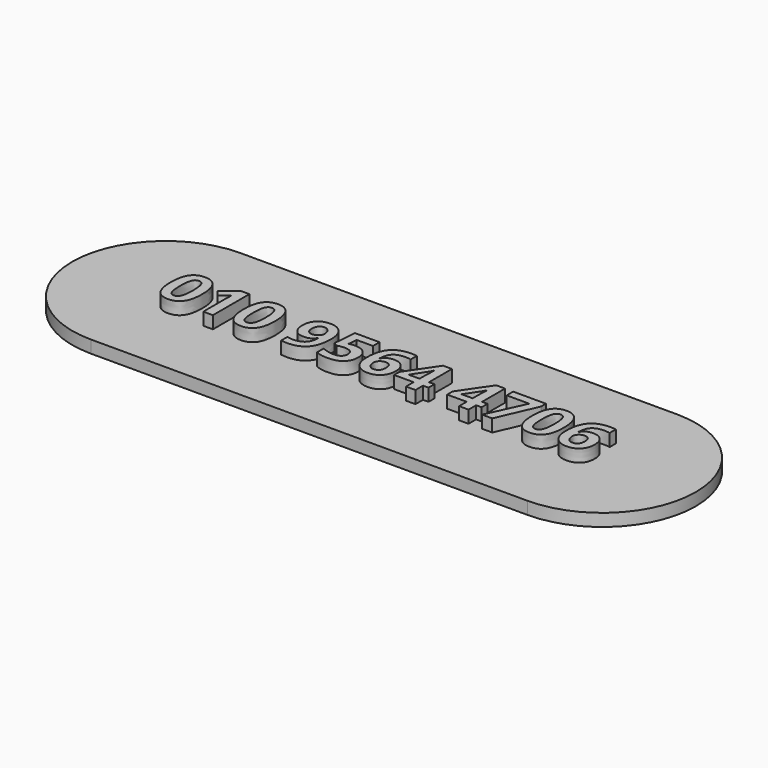
from build123d import *

# Parameters (mm, degrees)
F1_DEPTH     = 2
F2_TEXT_SIZE = 10.2467921594
F3_DEPTH     = 2


# Not quite as in the source:
# - Text() gives the source's letters only with a copy of the font that has no kerning and outlines rounded to 1/6400 em; it was checked with that copy


with BuildPart() as f1:
    # F0 (on Top) → F1 (new body)
    with BuildSketch(Plane.XY):
        with BuildLine():
            ThreePointArc((35, 15), (20, 0), (35, -15))
            Line((35, -15), (35, 15))
        make_face()
        with BuildLine():
            Line((-35, -15), (35, -15))
            ThreePointArc((35, -15), (20, 0), (35, 15))
            Line((35, 15), (-35, 15))
            ThreePointArc((-35, 15), (-24.3933982822, 10.6066017178), (-20, 0))
            ThreePointArc((-20, 0), (-24.3933982822, -10.6066017178), (-35, -15))
        make_face()
        with BuildLine():
            Line((35, 15), (35, -15))
            ThreePointArc((35, -15), (45.6066017178, -10.6066017178), (50, 0))
            ThreePointArc((50, 0), (45.6066017178, 10.6066017178), (35, 15))
        make_face()
        with BuildLine():
            ThreePointArc((-35, 15), (-50, 0), (-35, -15))
            Line((-35, -15), (-35, 15))
        make_face()
        with BuildLine():
            Line((-35, 15), (-35, -15))
            ThreePointArc((-35, -15), (-24.3933982822, -10.6066017178), (-20, 0))
            ThreePointArc((-20, 0), (-24.3933982822, 10.6066017178), (-35, 15))
        make_face()
    extrude(amount=-F1_DEPTH)

    # F2 (on face) → F3 (join)
    with BuildSketch(Plane.XY):
        with Locations((-34.8686458965, -3.3113568368)):
            Text('010 9564 4706', F2_TEXT_SIZE, font='Open Sans', font_style=FontStyle.BOLD, text_align=(TextAlign.LEFT, TextAlign.BOTTOM))
    extrude(amount=F3_DEPTH)


solid = f1.part
